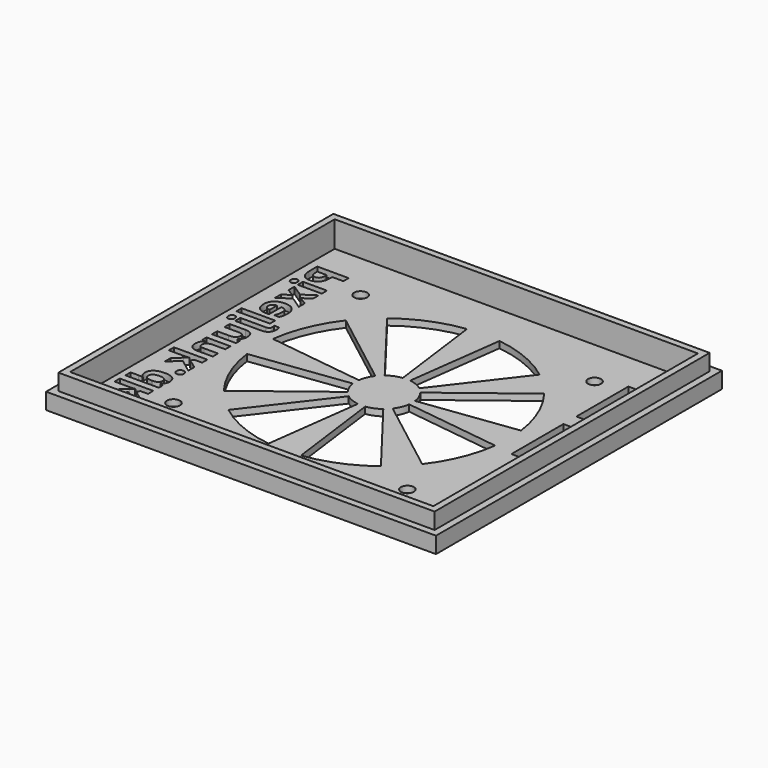
from build123d import *

# Parameters (mm, degrees)
F0_W          = 120
F0_H          = 110
F1_DEPTH      = 5
F2_W          = 115.8
F2_H          = 105.8
F3_DEPTH      = 5
F4_W          = 111.8
F4_H          = 101.8
F5_DEPTH      = 8
F6_R          = 2
F7_DEPTH      = 25
F8_W          = 9
F8_H          = 20
F9_DEPTH      = 25
F10_TEXT_SIZE = 13.5349981267
F11_DEPTH     = 25


# Not quite as in the source:
# - Text() gives the source's letters only with a copy of the font that has no kerning and outlines rounded to 1/6400 em; it was checked with that copy


with BuildPart() as f1:
    # F0 (on Top) → F1 (new body)
    with BuildSketch(Plane.XY):
        Rectangle(F0_W, F0_H)
    extrude(amount=F1_DEPTH)

    # F2 (on face) → F3 (join)
    with BuildSketch(Plane.XY.offset(5)):
        Rectangle(F2_W, F2_H)
    extrude(amount=F3_DEPTH)

    # F4 (on face) → F5 (cut)
    with BuildSketch(Plane.XY.offset(10)):
        Rectangle(F4_W, F4_H)
    extrude(amount=-F5_DEPTH, mode=Mode.SUBTRACT)

    # F6 (on face) → F7 (cut)
    with BuildSketch(Plane(origin=(0, 0, 0), x_dir=(1, 0, 0), z_dir=(0, 0, -1))):
        with BuildLine():
            ThreePointArc((-5.316902546, 6.9156793822), (-3.3382648227, 8.0592842098), (-1.1305059424, 8.6497416329))
            Line((-1.1305059424, 8.6497416329), (-4.9894474577, 38.1753246753))
            ThreePointArc((-4.9894474577, 38.1753246753), (-14.7333121461, 35.5693620017), (-23.4659588202, 30.5221030837))
            Line((-23.4659588202, 30.5221030837), (-5.316902546, 6.9156793822))
        make_face()
        with BuildLine():
            Line((5.316902546, 6.9156793822), (23.4659588202, 30.5221030837))
            ThreePointArc((23.4659588202, 30.5221030837), (14.7333121461, 35.5693620017), (4.9894474577, 38.1753246753))
            Line((4.9894474577, 38.1753246753), (1.1305059424, 8.6497416329))
            ThreePointArc((1.1305059424, 8.6497416329), (3.3382648227, 8.0592842098), (5.316902546, 6.9156793822))
        make_face()
        with BuildLine():
            Line((8.6497416329, 1.1305059424), (38.1753246753, 4.9894474577))
            ThreePointArc((38.1753246753, 4.9894474577), (35.5693620017, 14.7333121461), (30.5221030837, 23.4659588202))
            Line((30.5221030837, 23.4659588202), (6.9156793822, 5.316902546))
            ThreePointArc((6.9156793822, 5.316902546), (8.0592842098, 3.3382648227), (8.6497416329, 1.1305059424))
        make_face()
        with BuildLine():
            ThreePointArc((30.5221030837, -23.4659588202), (35.5693620017, -14.7333121461), (38.1753246753, -4.9894474577))
            Line((38.1753246753, -4.9894474577), (8.6497416329, -1.1305059424))
            ThreePointArc((8.6497416329, -1.1305059424), (8.0592842098, -3.3382648227), (6.9156793822, -5.316902546))
            Line((6.9156793822, -5.316902546), (30.5221030837, -23.4659588202))
        make_face()
        with BuildLine():
            ThreePointArc((4.9894474577, -38.1753246753), (14.7333121461, -35.5693620017), (23.4659588202, -30.5221030837))
            Line((23.4659588202, -30.5221030837), (5.316902546, -6.9156793822))
            ThreePointArc((5.316902546, -6.9156793822), (3.3382648227, -8.0592842098), (1.1305059424, -8.6497416329))
            Line((1.1305059424, -8.6497416329), (4.9894474577, -38.1753246753))
        make_face()
        with BuildLine():
            ThreePointArc((-1.1305059424, -8.6497416329), (-3.3382648227, -8.0592842098), (-5.316902546, -6.9156793822))
            Line((-5.316902546, -6.9156793822), (-23.4659588202, -30.5221030837))
            ThreePointArc((-23.4659588202, -30.5221030837), (-14.7333121461, -35.5693620017), (-4.9894474577, -38.1753246753))
            Line((-4.9894474577, -38.1753246753), (-1.1305059424, -8.6497416329))
        make_face()
        with BuildLine():
            ThreePointArc((-6.9156793822, -5.316902546), (-8.0592842098, -3.3382648227), (-8.6497416329, -1.1305059424))
            Line((-8.6497416329, -1.1305059424), (-38.1753246753, -4.9894474577))
            ThreePointArc((-38.1753246753, -4.9894474577), (-35.5693620017, -14.7333121461), (-30.5221030837, -23.4659588202))
            Line((-30.5221030837, -23.4659588202), (-6.9156793822, -5.316902546))
        make_face()
        with BuildLine():
            ThreePointArc((-8.6497416329, 1.1305059424), (-8.0592842098, 3.3382648227), (-6.9156793822, 5.316902546))
            Line((-6.9156793822, 5.316902546), (-30.5221030837, 23.4659588202))
            ThreePointArc((-30.5221030837, 23.4659588202), (-35.5693620017, 14.7333121461), (-38.1753246753, 4.9894474577))
            Line((-38.1753246753, 4.9894474577), (-8.6497416329, 1.1305059424))
        make_face()
        with Locations((36, 36)):
            Circle(F6_R)
        with Locations((-36, 36)):
            Circle(F6_R)
        with Locations((-36, -36)):
            Circle(F6_R)
        with Locations((36, -36)):
            Circle(F6_R)
    extrude(amount=-F7_DEPTH, mode=Mode.SUBTRACT)

    # F8 (on face) → F9 (cut)
    with BuildSketch(Plane(origin=(0, 0, 0), x_dir=(1, 0, 0), z_dir=(0, 0, -1))):
        with Locations((48.4999997616, -4)):
            Rectangle(F8_W, F8_H)
        with Locations((48.5, -29)):
            Rectangle(F8_W, F8_H)
    extrude(amount=-F9_DEPTH, mode=Mode.SUBTRACT)

    # F10 (on face) → F11 (cut)
    with BuildSketch(Plane(origin=(0, 0, 0), x_dir=(1, 0, 0), z_dir=(0, 0, -1))):
        with Locations(Location((-43.7432789867, -42.2958117241), (0, 0, 90))):
            Text('Pixeljunk.dk', F10_TEXT_SIZE, font='Open Sans', font_style=FontStyle.BOLD, text_align=(TextAlign.LEFT, TextAlign.BOTTOM))
    extrude(amount=-F11_DEPTH, mode=Mode.SUBTRACT)


solid = f1.part
